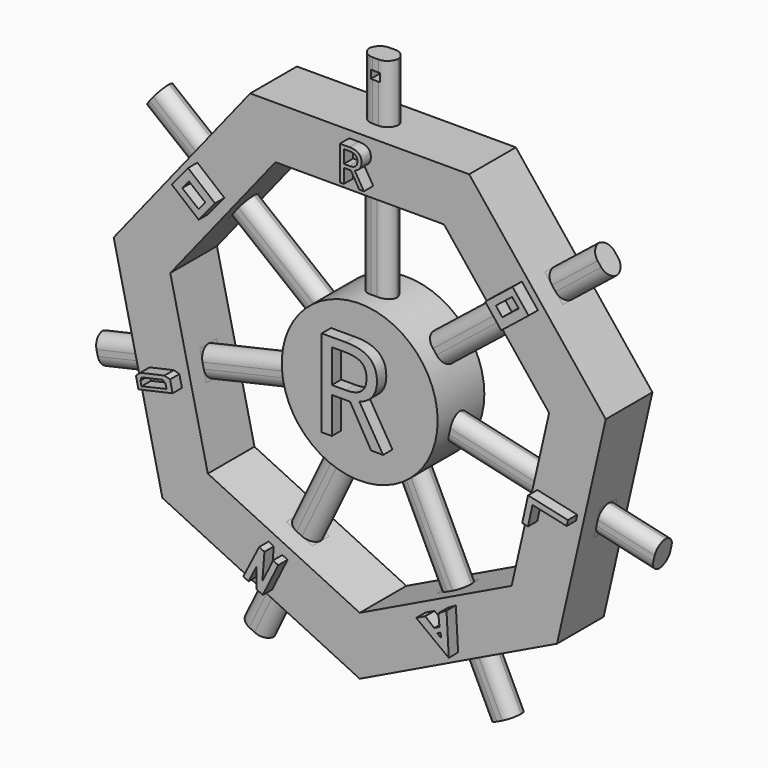
from build123d import *

# Parameters (mm, degrees)
F1_DEPTH      = 12.7
F7_W          = 6.35
F7_H          = 4.572
F9_DEPTH      = 25.4
F2_W          = 4.572
F2_H          = 6.35
F10_DEPTH     = 25.4
F4_W          = 6.35
F4_H          = 4.572
F11_DEPTH     = 25.4
F6_W          = 4.572
F6_H          = 6.35
F12_DEPTH     = 25.4
F3_W          = 6.35
F3_H          = 4.572
F13_DEPTH     = 25.4
F5_W          = 4.572
F5_H          = 6.35
F14_DEPTH     = 25.4
F8_W          = 4.572
F8_H          = 6.35
F15_DEPTH     = 25.4
F16_R         = 16.968135236
F17_DEPTH     = 12.7
F18_T4_DEPTH  = 27.8007641953
F18_S5_R      = 16.968135236
F18_T6_DEPTH  = 16
F18_T10_DEPTH = 27.7765131314
F18_S11_R     = 16.968135236
F18_T12_DEPTH = 16
F18_T16_DEPTH = 27.7765131314
F18_S17_R     = 16.968135236
F18_T18_DEPTH = 16
F18_T22_DEPTH = 27.8007641953
F18_S23_R     = 16.968135236
F18_T24_DEPTH = 16
F19_T4_DEPTH  = 27.7765131314
F19_S5_R      = 16.968135236
F19_T6_DEPTH  = 17
F19_T10_DEPTH = 27.8007641953
F19_S11_R     = 16.968135236
F19_T12_DEPTH = 17
F19_T16_DEPTH = 27.8007641953
F19_S17_R     = 16.968135236
F19_T18_DEPTH = 17
F19_T22_DEPTH = 27.7765131314
F19_S23_R     = 16.968135236
F19_T24_DEPTH = 17
F20_T4_DEPTH  = 27.7765131314
F20_S5_R      = 16.968135236
F20_T6_DEPTH  = 16
F20_T10_DEPTH = 27.8007641953
F20_S11_R     = 16.968135236
F20_T12_DEPTH = 16
F20_T16_DEPTH = 27.8007641953
F20_S17_R     = 16.968135236
F20_T18_DEPTH = 16
F20_T22_DEPTH = 27.7765131314
F20_S23_R     = 16.968135236
F20_T24_DEPTH = 16
F21_T4_DEPTH  = 27.8007641953
F21_S5_R      = 16.968135236
F21_T6_DEPTH  = 17
F21_T10_DEPTH = 27.7765131314
F21_S11_R     = 16.968135236
F21_T12_DEPTH = 17
F21_T16_DEPTH = 27.8007641953
F21_S17_R     = 16.968135236
F21_T18_DEPTH = 17
F21_T22_DEPTH = 27.7765131314
F21_S23_R     = 16.968135236
F21_T24_DEPTH = 17
F22_T4_DEPTH  = 27.8007641953
F22_S5_R      = 16.968135236
F22_T6_DEPTH  = 16
F22_T10_DEPTH = 27.7765131314
F22_S11_R     = 16.968135236
F22_T12_DEPTH = 16
F22_T16_DEPTH = 27.7765131314
F22_S17_R     = 16.968135236
F22_T18_DEPTH = 16
F22_T22_DEPTH = 27.8007641953
F22_S23_R     = 16.968135236
F22_T24_DEPTH = 16
F23_T4_DEPTH  = 27.8007641953
F23_S5_R      = 16.968135236
F23_T6_DEPTH  = 16
F23_T10_DEPTH = 27.7765131314
F23_S11_R     = 16.968135236
F23_T12_DEPTH = 16
F23_T16_DEPTH = 27.7765131314
F23_S17_R     = 16.968135236
F23_T18_DEPTH = 16
F23_T22_DEPTH = 27.8007641953
F23_S23_R     = 16.968135236
F23_T24_DEPTH = 16
F24_T4_DEPTH  = 27.8007641953
F24_S5_R      = 16.968135236
F24_T6_DEPTH  = 16
F24_T10_DEPTH = 27.7765131314
F24_S11_R     = 16.968135236
F24_T12_DEPTH = 16
F24_T16_DEPTH = 27.8007641953
F24_S17_R     = 16.968135236
F24_T18_DEPTH = 16
F24_T22_DEPTH = 27.7765131314
F24_S23_R     = 16.968135236
F24_T24_DEPTH = 16
F25_W         = 4.572
F25_H         = 6.35
F26_DEPTH     = 12.7
F32_W         = 4.572
F32_H         = 6.35
F33_DEPTH     = 12.7
F31_W         = 6.35
F31_H         = 4.572
F34_DEPTH     = 12.7
F30_W         = 4.572
F30_H         = 6.35
F35_DEPTH     = 12.7
F29_W         = 4.572
F29_H         = 6.35
F36_DEPTH     = 12.7
F28_W         = 6.35
F28_H         = 4.572
F37_DEPTH     = 12.7
F27_W         = 6.35
F27_H         = 4.572
F38_DEPTH     = 12.7
F39_T1_DEPTH  = 19.05
F40_T1_DEPTH  = 19.05
F41_T1_DEPTH  = 19.05
F42_T1_DEPTH  = 19.05
F43_T1_DEPTH  = 19.05
F44_T1_DEPTH  = 19.05
F45_T1_DEPTH  = 19.05
F46_W         = 0.3858066193
F46_H         = 1.778
F46_W_2       = 1.27
F46_W_3       = 0.3761933807
F47_DEPTH     = 25.4
F48_TEXT_SIZE = 26.5507492438
F49_DEPTH     = 2.54
F50_TEXT_SIZE = 26.5466622973
F51_DEPTH     = 2.54
F52_TEXT_SIZE = 10.4224828589
F53_DEPTH     = 2.54


# Not quite as in the source:
# - a fillet or chamfer that OpenCascade refuses, or shapes differently, is made with other operations: its cross-section is extruded or revolved along the edge and cut away or added
# - Text() gives the source's letters only with a copy of the font that has no kerning and outlines rounded to 1/6400 em; it was checked with that copy


with BuildPart() as f1:
    # F0 (on Front) → F1 (new body)
    with BuildSketch(Plane.XZ):
        Polygon((23.8356489691, 49.4952350855), (-23.8356489691, 49.4952350855), (-53.5582170749, 12.2243135473), (-42.9503553348, -34.2517654225), (0, -54.9355664205), (42.9503553348, -34.2517654225), (53.5582170749, 12.2243135473), align=None)
        Polygon((-41.2350925481, 9.41164079), (-18.3513426111, 38.1069555879), (18.3513426111, 38.1069555879), (41.2350925481, 9.41164079), (33.0679767537, -26.3708314853), (0, -42.2955297852), (-33.0679767537, -26.3708314853), align=None, mode=Mode.SUBTRACT)
    extrude(amount=F1_DEPTH)

    # F7 (on face) → F9 (join)
    with BuildSketch(Plane(origin=(0, 0, 38.1069555879), x_dir=(1, 0, 0), z_dir=(0, 0, -1))):
        with Locations((0.0636573889, 6.604)):
            Rectangle(F7_W, F7_H)
    extrude(amount=F9_DEPTH)

    # F2 (on face) → F10 (join)
    with BuildSketch(Plane(origin=(-37.1515346509, 0, -8.4795953476), x_dir=(0, 1, 0), z_dir=(0.9749279122, 0, 0.222520934))):
        with Locations((-6.604, -0.0636573889)):
            Rectangle(F2_W, F2_H)
    extrude(amount=F10_DEPTH)

    # F4 (on face) → F11 (join)
    with BuildSketch(Plane(origin=(16.5339883768, 0, -34.3331806352), x_dir=(0.9009688679, 0, 0.4338837391), z_dir=(-0.4338837391, 0, 0.9009688679))):
        with Locations((0.0636573889, -6.604)):
            Rectangle(F4_W, F4_H)
    extrude(amount=F11_DEPTH)

    # F6 (on face) → F12 (join)
    with BuildSketch(Plane(origin=(29.7932175796, 0, 23.7592981889), x_dir=(0, -1, 0), z_dir=(-0.7818314825, 0, -0.6234898019))):
        with Locations((6.604, -0.0636573889)):
            Rectangle(F6_W, F6_H)
    extrude(amount=F12_DEPTH)

    # F3 (on face) → F13 (join)
    with BuildSketch(Plane(origin=(-16.5339883768, 0, -34.3331806352), x_dir=(0.9009688679, 0, -0.4338837391), z_dir=(0.4338837391, 0, 0.9009688679))):
        with Locations((-0.0636573889, -6.096)):
            Rectangle(F3_W, F3_H)
    extrude(amount=F13_DEPTH)

    # F5 (on face) → F14 (join)
    with BuildSketch(Plane(origin=(37.1515346509, 0, -8.4795953476), x_dir=(0, -1, 0), z_dir=(-0.9749279122, 0, 0.222520934))):
        with Locations((6.604, 0.0636573889)):
            Rectangle(F5_W, F5_H)
    extrude(amount=F14_DEPTH)

    # F8 (on face) → F15 (join)
    with BuildSketch(Plane(origin=(-29.7932175796, 0, 23.7592981889), x_dir=(0, 1, 0), z_dir=(0.7818314825, 0, -0.6234898019))):
        with Locations((-6.604, -0.0636573889)):
            Rectangle(F8_W, F8_H)
    extrude(amount=F15_DEPTH)

    # F16 (on Front) → F17 (join)
    with BuildSketch(Plane.XZ):
        Circle(F16_R)
    extrude(amount=F17_DEPTH)

    # F18: fillet of radius 2.54 on 4 edges, made by hand


with BuildPart() as f18_tool2:
    # F18_s3 → F18_t4 (new body)
    with BuildSketch(Plane(origin=(37.1515346509, 0, -8.4795953476), x_dir=(0, 1, 0), z_dir=(-0.9749279122, 0, 0.222520934))):
        with BuildLine():
            ThreePointArc((-6.35, -3.2386573889), (-8.1460512242, -2.4947086131), (-8.89, -0.6986573889))
            Line((-8.89, -0.6986573889), (-8.89, -3.2386573889))
            Line((-8.89, -3.2386573889), (-6.35, -3.2386573889))
        make_face()
    extrude(amount=F18_T4_DEPTH)

    # F18_s5 → F18_t6 (cut, symmetric)
    with BuildSketch(Plane.XZ.offset(7.6)):
        Circle(F18_S5_R)
    extrude(amount=F18_T6_DEPTH, both=True, mode=Mode.SUBTRACT)


with BuildPart() as f1_1:
    add(f1.part)

    # F18_t1: cut F18_tool2
    add(f18_tool2.part, mode=Mode.SUBTRACT)


with BuildPart() as f18_tool8:
    # F18_s9 → F18_t10 (new body)
    with BuildSketch(Plane(origin=(37.1515346509, 0, -8.4795953476), x_dir=(0, 1, 0), z_dir=(-0.9749279122, 0, 0.222520934))):
        with BuildLine():
            ThreePointArc((-4.318, 0.5713426111), (-5.0619487758, 2.3673938354), (-6.858, 3.1113426111))
            Line((-6.858, 3.1113426111), (-4.318, 3.1113426111))
            Line((-4.318, 3.1113426111), (-4.318, 0.5713426111))
        make_face()
    extrude(amount=F18_T10_DEPTH)

    # F18_s11 → F18_t12 (cut, symmetric)
    with BuildSketch(Plane.XZ.offset(5.6)):
        Circle(F18_S11_R)
    extrude(amount=F18_T12_DEPTH, both=True, mode=Mode.SUBTRACT)


with BuildPart() as f1_2:
    add(f1_1.part)

    # F18_t7: cut F18_tool8
    add(f18_tool8.part, mode=Mode.SUBTRACT)


with BuildPart() as f18_tool14:
    # F18_s15 → F18_t16 (new body)
    with BuildSketch(Plane(origin=(37.1515346509, 0, -8.4795953476), x_dir=(0, 1, 0), z_dir=(-0.9749279122, 0, 0.222520934))):
        with BuildLine():
            ThreePointArc((-8.89, 0.5713426111), (-8.1460512242, 2.3673938354), (-6.35, 3.1113426111))
            Line((-6.35, 3.1113426111), (-8.89, 3.1113426111))
            Line((-8.89, 3.1113426111), (-8.89, 0.5713426111))
        make_face()
    extrude(amount=F18_T16_DEPTH)

    # F18_s17 → F18_t18 (cut, symmetric)
    with BuildSketch(Plane.XZ.offset(7.6)):
        Circle(F18_S17_R)
    extrude(amount=F18_T18_DEPTH, both=True, mode=Mode.SUBTRACT)


with BuildPart() as f1_3:
    add(f1_2.part)

    # F18_t13: cut F18_tool14
    add(f18_tool14.part, mode=Mode.SUBTRACT)


with BuildPart() as f18_tool20:
    # F18_s21 → F18_t22 (new body)
    with BuildSketch(Plane(origin=(37.1515346509, 0, -8.4795953476), x_dir=(0, 1, 0), z_dir=(-0.9749279122, 0, 0.222520934))):
        with BuildLine():
            ThreePointArc((-4.318, -0.6986573889), (-5.0619487758, -2.4947086131), (-6.858, -3.2386573889))
            Line((-6.858, -3.2386573889), (-4.318, -3.2386573889))
            Line((-4.318, -3.2386573889), (-4.318, -0.6986573889))
        make_face()
    extrude(amount=F18_T22_DEPTH)

    # F18_s23 → F18_t24 (cut, symmetric)
    with BuildSketch(Plane.XZ.offset(5.6)):
        Circle(F18_S23_R)
    extrude(amount=F18_T24_DEPTH, both=True, mode=Mode.SUBTRACT)


with BuildPart() as f1_4:
    add(f1_3.part)

    # F18_t19: cut F18_tool20
    add(f18_tool20.part, mode=Mode.SUBTRACT)

    # F19: fillet of radius 2.54 on 4 edges, made by hand


with BuildPart() as f19_tool2:
    # F19_s3 → F19_t4 (new body)
    with BuildSketch(Plane(origin=(29.7932175796, 0, 23.7592981889), x_dir=(0, 1, 0), z_dir=(-0.7818314825, 0, -0.6234898019))):
        with BuildLine():
            ThreePointArc((-8.89, -0.5713426111), (-8.1460512242, -2.3673938354), (-6.35, -3.1113426111))
            Line((-6.35, -3.1113426111), (-8.89, -3.1113426111))
            Line((-8.89, -3.1113426111), (-8.89, -0.5713426111))
        make_face()
    extrude(amount=F19_T4_DEPTH)

    # F19_s5 → F19_t6 (cut, symmetric)
    with BuildSketch(Plane.XZ.offset(7.6)):
        Circle(F19_S5_R)
    extrude(amount=F19_T6_DEPTH, both=True, mode=Mode.SUBTRACT)


with BuildPart() as f1_5:
    add(f1_4.part)

    # F19_t1: cut F19_tool2
    add(f19_tool2.part, mode=Mode.SUBTRACT)


with BuildPart() as f19_tool8:
    # F19_s9 → F19_t10 (new body)
    with BuildSketch(Plane(origin=(29.7932175796, 0, 23.7592981889), x_dir=(0, 1, 0), z_dir=(-0.7818314825, 0, -0.6234898019))):
        with BuildLine():
            ThreePointArc((-6.35, 3.2386573889), (-8.1460512242, 2.4947086131), (-8.89, 0.6986573889))
            Line((-8.89, 0.6986573889), (-8.89, 3.2386573889))
            Line((-8.89, 3.2386573889), (-6.35, 3.2386573889))
        make_face()
    extrude(amount=F19_T10_DEPTH)

    # F19_s11 → F19_t12 (cut, symmetric)
    with BuildSketch(Plane.XZ.offset(7.6)):
        Circle(F19_S11_R)
    extrude(amount=F19_T12_DEPTH, both=True, mode=Mode.SUBTRACT)


with BuildPart() as f1_6:
    add(f1_5.part)

    # F19_t7: cut F19_tool8
    add(f19_tool8.part, mode=Mode.SUBTRACT)


with BuildPart() as f19_tool14:
    # F19_s15 → F19_t16 (new body)
    with BuildSketch(Plane(origin=(29.7932175796, 0, 23.7592981889), x_dir=(0, 1, 0), z_dir=(-0.7818314825, 0, -0.6234898019))):
        with BuildLine():
            ThreePointArc((-4.318, 0.6986573889), (-5.0619487758, 2.4947086131), (-6.858, 3.2386573889))
            Line((-6.858, 3.2386573889), (-4.318, 3.2386573889))
            Line((-4.318, 3.2386573889), (-4.318, 0.6986573889))
        make_face()
    extrude(amount=F19_T16_DEPTH)

    # F19_s17 → F19_t18 (cut, symmetric)
    with BuildSketch(Plane.XZ.offset(5.6)):
        Circle(F19_S17_R)
    extrude(amount=F19_T18_DEPTH, both=True, mode=Mode.SUBTRACT)


with BuildPart() as f1_7:
    add(f1_6.part)

    # F19_t13: cut F19_tool14
    add(f19_tool14.part, mode=Mode.SUBTRACT)


with BuildPart() as f19_tool20:
    # F19_s21 → F19_t22 (new body)
    with BuildSketch(Plane(origin=(29.7932175796, 0, 23.7592981889), x_dir=(0, 1, 0), z_dir=(-0.7818314825, 0, -0.6234898019))):
        with BuildLine():
            ThreePointArc((-4.318, -0.5713426111), (-5.0619487758, -2.3673938354), (-6.858, -3.1113426111))
            Line((-6.858, -3.1113426111), (-4.318, -3.1113426111))
            Line((-4.318, -3.1113426111), (-4.318, -0.5713426111))
        make_face()
    extrude(amount=F19_T22_DEPTH)

    # F19_s23 → F19_t24 (cut, symmetric)
    with BuildSketch(Plane.XZ.offset(5.6)):
        Circle(F19_S23_R)
    extrude(amount=F19_T24_DEPTH, both=True, mode=Mode.SUBTRACT)


with BuildPart() as f1_8:
    add(f1_7.part)

    # F19_t19: cut F19_tool20
    add(f19_tool20.part, mode=Mode.SUBTRACT)

    # F20: fillet of radius 2.54 on 4 edges, made by hand


with BuildPart() as f20_tool2:
    # F20_s3 → F20_t4 (new body)
    with BuildSketch(Plane.XY.offset(38.1069555879)):
        with BuildLine():
            ThreePointArc((-0.5713426111, -8.89), (-2.3673938354, -8.1460512242), (-3.1113426111, -6.35))
            Line((-3.1113426111, -6.35), (-3.1113426111, -8.89))
            Line((-3.1113426111, -8.89), (-0.5713426111, -8.89))
        make_face()
    extrude(amount=-F20_T4_DEPTH)

    # F20_s5 → F20_t6 (cut, symmetric)
    with BuildSketch(Plane.XZ.offset(7.6)):
        Circle(F20_S5_R)
    extrude(amount=F20_T6_DEPTH, both=True, mode=Mode.SUBTRACT)


with BuildPart() as f1_9:
    add(f1_8.part)

    # F20_t1: cut F20_tool2
    add(f20_tool2.part, mode=Mode.SUBTRACT)


with BuildPart() as f20_tool8:
    # F20_s9 → F20_t10 (new body)
    with BuildSketch(Plane.XY.offset(38.1069555879)):
        with BuildLine():
            ThreePointArc((0.6986573889, -4.318), (2.4947086131, -5.0619487758), (3.2386573889, -6.858))
            Line((3.2386573889, -6.858), (3.2386573889, -4.318))
            Line((3.2386573889, -4.318), (0.6986573889, -4.318))
        make_face()
    extrude(amount=-F20_T10_DEPTH)

    # F20_s11 → F20_t12 (cut, symmetric)
    with BuildSketch(Plane.XZ.offset(5.6)):
        Circle(F20_S11_R)
    extrude(amount=F20_T12_DEPTH, both=True, mode=Mode.SUBTRACT)


with BuildPart() as f1_10:
    add(f1_9.part)

    # F20_t7: cut F20_tool8
    add(f20_tool8.part, mode=Mode.SUBTRACT)


with BuildPart() as f20_tool14:
    # F20_s15 → F20_t16 (new body)
    with BuildSketch(Plane.XY.offset(38.1069555879)):
        with BuildLine():
            ThreePointArc((3.2386573889, -6.35), (2.4947086131, -8.1460512242), (0.6986573889, -8.89))
            Line((0.6986573889, -8.89), (3.2386573889, -8.89))
            Line((3.2386573889, -8.89), (3.2386573889, -6.35))
        make_face()
    extrude(amount=-F20_T16_DEPTH)

    # F20_s17 → F20_t18 (cut, symmetric)
    with BuildSketch(Plane.XZ.offset(7.6)):
        Circle(F20_S17_R)
    extrude(amount=F20_T18_DEPTH, both=True, mode=Mode.SUBTRACT)


with BuildPart() as f1_11:
    add(f1_10.part)

    # F20_t13: cut F20_tool14
    add(f20_tool14.part, mode=Mode.SUBTRACT)


with BuildPart() as f20_tool20:
    # F20_s21 → F20_t22 (new body)
    with BuildSketch(Plane.XY.offset(38.1069555879)):
        with BuildLine():
            ThreePointArc((-0.5713426111, -4.318), (-2.3673938354, -5.0619487758), (-3.1113426111, -6.858))
            Line((-3.1113426111, -6.858), (-3.1113426111, -4.318))
            Line((-3.1113426111, -4.318), (-0.5713426111, -4.318))
        make_face()
    extrude(amount=-F20_T22_DEPTH)

    # F20_s23 → F20_t24 (cut, symmetric)
    with BuildSketch(Plane.XZ.offset(5.6)):
        Circle(F20_S23_R)
    extrude(amount=F20_T24_DEPTH, both=True, mode=Mode.SUBTRACT)


with BuildPart() as f1_12:
    add(f1_11.part)

    # F20_t19: cut F20_tool20
    add(f20_tool20.part, mode=Mode.SUBTRACT)

    # F21: fillet of radius 2.54 on 4 edges, made by hand


with BuildPart() as f21_tool2:
    # F21_s3 → F21_t4 (new body)
    with BuildSketch(Plane(origin=(-29.7932175796, 0, 23.7592981889), x_dir=(0, 1, 0), z_dir=(0.7818314825, 0, -0.6234898019))):
        with BuildLine():
            ThreePointArc((-4.318, -0.6986573889), (-5.0619487758, -2.4947086131), (-6.858, -3.2386573889))
            Line((-6.858, -3.2386573889), (-4.318, -3.2386573889))
            Line((-4.318, -3.2386573889), (-4.318, -0.6986573889))
        make_face()
    extrude(amount=F21_T4_DEPTH)

    # F21_s5 → F21_t6 (cut, symmetric)
    with BuildSketch(Plane.XZ.offset(5.6)):
        Circle(F21_S5_R)
    extrude(amount=F21_T6_DEPTH, both=True, mode=Mode.SUBTRACT)


with BuildPart() as f1_13:
    add(f1_12.part)

    # F21_t1: cut F21_tool2
    add(f21_tool2.part, mode=Mode.SUBTRACT)


with BuildPart() as f21_tool8:
    # F21_s9 → F21_t10 (new body)
    with BuildSketch(Plane(origin=(-29.7932175796, 0, 23.7592981889), x_dir=(0, 1, 0), z_dir=(0.7818314825, 0, -0.6234898019))):
        with BuildLine():
            ThreePointArc((-4.318, 0.5713426111), (-5.0619487758, 2.3673938354), (-6.858, 3.1113426111))
            Line((-6.858, 3.1113426111), (-4.318, 3.1113426111))
            Line((-4.318, 3.1113426111), (-4.318, 0.5713426111))
        make_face()
    extrude(amount=F21_T10_DEPTH)

    # F21_s11 → F21_t12 (cut, symmetric)
    with BuildSketch(Plane.XZ.offset(5.6)):
        Circle(F21_S11_R)
    extrude(amount=F21_T12_DEPTH, both=True, mode=Mode.SUBTRACT)


with BuildPart() as f1_14:
    add(f1_13.part)

    # F21_t7: cut F21_tool8
    add(f21_tool8.part, mode=Mode.SUBTRACT)


with BuildPart() as f21_tool14:
    # F21_s15 → F21_t16 (new body)
    with BuildSketch(Plane(origin=(-29.7932175796, 0, 23.7592981889), x_dir=(0, 1, 0), z_dir=(0.7818314825, 0, -0.6234898019))):
        with BuildLine():
            ThreePointArc((-8.89, -0.6986573889), (-8.1460512242, -2.4947086131), (-6.35, -3.2386573889))
            Line((-6.35, -3.2386573889), (-8.89, -3.2386573889))
            Line((-8.89, -3.2386573889), (-8.89, -0.6986573889))
        make_face()
    extrude(amount=F21_T16_DEPTH)

    # F21_s17 → F21_t18 (cut, symmetric)
    with BuildSketch(Plane.XZ.offset(7.6)):
        Circle(F21_S17_R)
    extrude(amount=F21_T18_DEPTH, both=True, mode=Mode.SUBTRACT)


with BuildPart() as f1_15:
    add(f1_14.part)

    # F21_t13: cut F21_tool14
    add(f21_tool14.part, mode=Mode.SUBTRACT)


with BuildPart() as f21_tool20:
    # F21_s21 → F21_t22 (new body)
    with BuildSketch(Plane(origin=(-29.7932175796, 0, 23.7592981889), x_dir=(0, 1, 0), z_dir=(0.7818314825, 0, -0.6234898019))):
        with BuildLine():
            ThreePointArc((-6.35, 3.1113426111), (-8.1460512242, 2.3673938354), (-8.89, 0.5713426111))
            Line((-8.89, 0.5713426111), (-8.89, 3.1113426111))
            Line((-8.89, 3.1113426111), (-6.35, 3.1113426111))
        make_face()
    extrude(amount=F21_T22_DEPTH)

    # F21_s23 → F21_t24 (cut, symmetric)
    with BuildSketch(Plane.XZ.offset(7.6)):
        Circle(F21_S23_R)
    extrude(amount=F21_T24_DEPTH, both=True, mode=Mode.SUBTRACT)


with BuildPart() as f1_16:
    add(f1_15.part)

    # F21_t19: cut F21_tool20
    add(f21_tool20.part, mode=Mode.SUBTRACT)

    # F22: fillet of radius 2.54 on 4 edges, made by hand


with BuildPart() as f22_tool2:
    # F22_s3 → F22_t4 (new body)
    with BuildSketch(Plane(origin=(-37.1515346509, 0, -8.4795953476), x_dir=(0, 1, 0), z_dir=(0.9749279122, 0, 0.222520934))):
        with BuildLine():
            ThreePointArc((-4.318, -0.6986573889), (-5.0619487758, -2.4947086131), (-6.858, -3.2386573889))
            Line((-6.858, -3.2386573889), (-4.318, -3.2386573889))
            Line((-4.318, -3.2386573889), (-4.318, -0.6986573889))
        make_face()
    extrude(amount=F22_T4_DEPTH)

    # F22_s5 → F22_t6 (cut, symmetric)
    with BuildSketch(Plane.XZ.offset(5.6)):
        Circle(F22_S5_R)
    extrude(amount=F22_T6_DEPTH, both=True, mode=Mode.SUBTRACT)


with BuildPart() as f1_17:
    add(f1_16.part)

    # F22_t1: cut F22_tool2
    add(f22_tool2.part, mode=Mode.SUBTRACT)


with BuildPart() as f22_tool8:
    # F22_s9 → F22_t10 (new body)
    with BuildSketch(Plane(origin=(-37.1515346509, 0, -8.4795953476), x_dir=(0, 1, 0), z_dir=(0.9749279122, 0, 0.222520934))):
        with BuildLine():
            ThreePointArc((-4.318, 0.5713426111), (-5.0619487758, 2.3673938354), (-6.858, 3.1113426111))
            Line((-6.858, 3.1113426111), (-4.318, 3.1113426111))
            Line((-4.318, 3.1113426111), (-4.318, 0.5713426111))
        make_face()
    extrude(amount=F22_T10_DEPTH)

    # F22_s11 → F22_t12 (cut, symmetric)
    with BuildSketch(Plane.XZ.offset(5.6)):
        Circle(F22_S11_R)
    extrude(amount=F22_T12_DEPTH, both=True, mode=Mode.SUBTRACT)


with BuildPart() as f1_18:
    add(f1_17.part)

    # F22_t7: cut F22_tool8
    add(f22_tool8.part, mode=Mode.SUBTRACT)


with BuildPart() as f22_tool14:
    # F22_s15 → F22_t16 (new body)
    with BuildSketch(Plane(origin=(-37.1515346509, 0, -8.4795953476), x_dir=(0, 1, 0), z_dir=(0.9749279122, 0, 0.222520934))):
        with BuildLine():
            ThreePointArc((-8.89, 0.5713426111), (-8.1460512242, 2.3673938354), (-6.35, 3.1113426111))
            Line((-6.35, 3.1113426111), (-8.89, 3.1113426111))
            Line((-8.89, 3.1113426111), (-8.89, 0.5713426111))
        make_face()
    extrude(amount=F22_T16_DEPTH)

    # F22_s17 → F22_t18 (cut, symmetric)
    with BuildSketch(Plane.XZ.offset(7.6)):
        Circle(F22_S17_R)
    extrude(amount=F22_T18_DEPTH, both=True, mode=Mode.SUBTRACT)


with BuildPart() as f1_19:
    add(f1_18.part)

    # F22_t13: cut F22_tool14
    add(f22_tool14.part, mode=Mode.SUBTRACT)


with BuildPart() as f22_tool20:
    # F22_s21 → F22_t22 (new body)
    with BuildSketch(Plane(origin=(-37.1515346509, 0, -8.4795953476), x_dir=(0, 1, 0), z_dir=(0.9749279122, 0, 0.222520934))):
        with BuildLine():
            ThreePointArc((-6.35, -3.2386573889), (-8.1460512242, -2.4947086131), (-8.89, -0.6986573889))
            Line((-8.89, -0.6986573889), (-8.89, -3.2386573889))
            Line((-8.89, -3.2386573889), (-6.35, -3.2386573889))
        make_face()
    extrude(amount=F22_T22_DEPTH)

    # F22_s23 → F22_t24 (cut, symmetric)
    with BuildSketch(Plane.XZ.offset(7.6)):
        Circle(F22_S23_R)
    extrude(amount=F22_T24_DEPTH, both=True, mode=Mode.SUBTRACT)


with BuildPart() as f1_20:
    add(f1_19.part)

    # F22_t19: cut F22_tool20
    add(f22_tool20.part, mode=Mode.SUBTRACT)

    # F23: fillet of radius 2.54 on 4 edges, made by hand


with BuildPart() as f23_tool2:
    # F23_s3 → F23_t4 (new body)
    with BuildSketch(Plane(origin=(-16.5339883768, 0, -34.3331806352), x_dir=(0, 1, 0), z_dir=(0.4338837391, 0, 0.9009688679))):
        with BuildLine():
            ThreePointArc((-6.35, 3.2386573889), (-4.5539487758, 2.4947086131), (-3.81, 0.6986573889))
            Line((-3.81, 0.6986573889), (-3.81, 3.2386573889))
            Line((-3.81, 3.2386573889), (-6.35, 3.2386573889))
        make_face()
    extrude(amount=F23_T4_DEPTH)

    # F23_s5 → F23_t6 (cut, symmetric)
    with BuildSketch(Plane.XZ.offset(5.1)):
        Circle(F23_S5_R)
    extrude(amount=F23_T6_DEPTH, both=True, mode=Mode.SUBTRACT)


with BuildPart() as f1_21:
    add(f1_20.part)

    # F23_t1: cut F23_tool2
    add(f23_tool2.part, mode=Mode.SUBTRACT)


with BuildPart() as f23_tool8:
    # F23_s9 → F23_t10 (new body)
    with BuildSketch(Plane(origin=(-16.5339883768, 0, -34.3331806352), x_dir=(0, 1, 0), z_dir=(0.4338837391, 0, 0.9009688679))):
        with BuildLine():
            ThreePointArc((-6.35, -3.1113426111), (-4.5539487758, -2.3673938354), (-3.81, -0.5713426111))
            Line((-3.81, -0.5713426111), (-3.81, -3.1113426111))
            Line((-3.81, -3.1113426111), (-6.35, -3.1113426111))
        make_face()
    extrude(amount=F23_T10_DEPTH)

    # F23_s11 → F23_t12 (cut, symmetric)
    with BuildSketch(Plane.XZ.offset(5.1)):
        Circle(F23_S11_R)
    extrude(amount=F23_T12_DEPTH, both=True, mode=Mode.SUBTRACT)


with BuildPart() as f1_22:
    add(f1_21.part)

    # F23_t7: cut F23_tool8
    add(f23_tool8.part, mode=Mode.SUBTRACT)


with BuildPart() as f23_tool14:
    # F23_s15 → F23_t16 (new body)
    with BuildSketch(Plane(origin=(-16.5339883768, 0, -34.3331806352), x_dir=(0, 1, 0), z_dir=(0.4338837391, 0, 0.9009688679))):
        with BuildLine():
            ThreePointArc((-8.382, -0.5713426111), (-7.6380512242, -2.3673938354), (-5.842, -3.1113426111))
            Line((-5.842, -3.1113426111), (-8.382, -3.1113426111))
            Line((-8.382, -3.1113426111), (-8.382, -0.5713426111))
        make_face()
    extrude(amount=F23_T16_DEPTH)

    # F23_s17 → F23_t18 (cut, symmetric)
    with BuildSketch(Plane.XZ.offset(7.1)):
        Circle(F23_S17_R)
    extrude(amount=F23_T18_DEPTH, both=True, mode=Mode.SUBTRACT)


with BuildPart() as f1_23:
    add(f1_22.part)

    # F23_t13: cut F23_tool14
    add(f23_tool14.part, mode=Mode.SUBTRACT)


with BuildPart() as f23_tool20:
    # F23_s21 → F23_t22 (new body)
    with BuildSketch(Plane(origin=(-16.5339883768, 0, -34.3331806352), x_dir=(0, 1, 0), z_dir=(0.4338837391, 0, 0.9009688679))):
        with BuildLine():
            ThreePointArc((-5.842, 3.2386573889), (-7.6380512242, 2.4947086131), (-8.382, 0.6986573889))
            Line((-8.382, 0.6986573889), (-8.382, 3.2386573889))
            Line((-8.382, 3.2386573889), (-5.842, 3.2386573889))
        make_face()
    extrude(amount=F23_T22_DEPTH)

    # F23_s23 → F23_t24 (cut, symmetric)
    with BuildSketch(Plane.XZ.offset(7.1)):
        Circle(F23_S23_R)
    extrude(amount=F23_T24_DEPTH, both=True, mode=Mode.SUBTRACT)


with BuildPart() as f1_24:
    add(f1_23.part)

    # F23_t19: cut F23_tool20
    add(f23_tool20.part, mode=Mode.SUBTRACT)

    # F24: fillet of radius 2.54 on 4 edges, made by hand


with BuildPart() as f24_tool2:
    # F24_s3 → F24_t4 (new body)
    with BuildSketch(Plane(origin=(16.5339883768, 0, -34.3331806352), x_dir=(0, 1, 0), z_dir=(-0.4338837391, 0, 0.9009688679))):
        with BuildLine():
            ThreePointArc((-6.858, -3.2386573889), (-5.0619487758, -2.4947086131), (-4.318, -0.6986573889))
            Line((-4.318, -0.6986573889), (-4.318, -3.2386573889))
            Line((-4.318, -3.2386573889), (-6.858, -3.2386573889))
        make_face()
    extrude(amount=F24_T4_DEPTH)

    # F24_s5 → F24_t6 (cut, symmetric)
    with BuildSketch(Plane.XZ.offset(5.6)):
        Circle(F24_S5_R)
    extrude(amount=F24_T6_DEPTH, both=True, mode=Mode.SUBTRACT)


with BuildPart() as f1_25:
    add(f1_24.part)

    # F24_t1: cut F24_tool2
    add(f24_tool2.part, mode=Mode.SUBTRACT)


with BuildPart() as f24_tool8:
    # F24_s9 → F24_t10 (new body)
    with BuildSketch(Plane(origin=(16.5339883768, 0, -34.3331806352), x_dir=(0, 1, 0), z_dir=(-0.4338837391, 0, 0.9009688679))):
        with BuildLine():
            ThreePointArc((-6.858, 3.1113426111), (-5.0619487758, 2.3673938354), (-4.318, 0.5713426111))
            Line((-4.318, 0.5713426111), (-4.318, 3.1113426111))
            Line((-4.318, 3.1113426111), (-6.858, 3.1113426111))
        make_face()
    extrude(amount=F24_T10_DEPTH)

    # F24_s11 → F24_t12 (cut, symmetric)
    with BuildSketch(Plane.XZ.offset(5.6)):
        Circle(F24_S11_R)
    extrude(amount=F24_T12_DEPTH, both=True, mode=Mode.SUBTRACT)


with BuildPart() as f1_26:
    add(f1_25.part)

    # F24_t7: cut F24_tool8
    add(f24_tool8.part, mode=Mode.SUBTRACT)


with BuildPart() as f24_tool14:
    # F24_s15 → F24_t16 (new body)
    with BuildSketch(Plane(origin=(16.5339883768, 0, -34.3331806352), x_dir=(0, 1, 0), z_dir=(-0.4338837391, 0, 0.9009688679))):
        with BuildLine():
            ThreePointArc((-6.35, -3.2386573889), (-8.1460512242, -2.4947086131), (-8.89, -0.6986573889))
            Line((-8.89, -0.6986573889), (-8.89, -3.2386573889))
            Line((-8.89, -3.2386573889), (-6.35, -3.2386573889))
        make_face()
    extrude(amount=F24_T16_DEPTH)

    # F24_s17 → F24_t18 (cut, symmetric)
    with BuildSketch(Plane.XZ.offset(7.6)):
        Circle(F24_S17_R)
    extrude(amount=F24_T18_DEPTH, both=True, mode=Mode.SUBTRACT)


with BuildPart() as f1_27:
    add(f1_26.part)

    # F24_t13: cut F24_tool14
    add(f24_tool14.part, mode=Mode.SUBTRACT)


with BuildPart() as f24_tool20:
    # F24_s21 → F24_t22 (new body)
    with BuildSketch(Plane(origin=(16.5339883768, 0, -34.3331806352), x_dir=(0, 1, 0), z_dir=(-0.4338837391, 0, 0.9009688679))):
        with BuildLine():
            ThreePointArc((-8.89, 0.5713426111), (-8.1460512242, 2.3673938354), (-6.35, 3.1113426111))
            Line((-6.35, 3.1113426111), (-8.89, 3.1113426111))
            Line((-8.89, 3.1113426111), (-8.89, 0.5713426111))
        make_face()
    extrude(amount=F24_T22_DEPTH)

    # F24_s23 → F24_t24 (cut, symmetric)
    with BuildSketch(Plane.XZ.offset(7.6)):
        Circle(F24_S23_R)
    extrude(amount=F24_T24_DEPTH, both=True, mode=Mode.SUBTRACT)


with BuildPart() as f1_28:
    add(f1_27.part)

    # F24_t19: cut F24_tool20
    add(f24_tool20.part, mode=Mode.SUBTRACT)

    # F25 (on face) → F26 (join)
    with BuildSketch(Plane(origin=(-48.2542862048, 0, -11.0137259376), x_dir=(0, -1, 0), z_dir=(-0.9749279122, 0, -0.222520934))):
        with Locations((6.096, -0.12286896)):
            Rectangle(F25_W, F25_H)
    extrude(amount=F26_DEPTH)

    # F32 (on face) → F33 (join)
    with BuildSketch(Plane(origin=(-38.696933022, 0, 30.8597743164), x_dir=(0, -1, 0), z_dir=(-0.7818314825, 0, 0.6234898019))):
        with Locations((6.096, -0.2494668204)):
            Rectangle(F32_W, F32_H)
    extrude(amount=F33_DEPTH)

    # F31 (on face) → F34 (join)
    with BuildSketch(Plane.XY.offset(49.4952350855)):
        with Locations((-0.0392214861, -6.096)):
            Rectangle(F31_W, F31_H)
    extrude(amount=F34_DEPTH)

    # F30 (on face) → F35 (join)
    with BuildSketch(Plane(origin=(38.696933022, 0, 30.8597743164), x_dir=(0, 1, 0), z_dir=(0.7818314825, 0, 0.6234898019))):
        with Locations((-6.096, -0.1651499968)):
            Rectangle(F30_W, F30_H)
    extrude(amount=F35_DEPTH)

    # F29 (on face) → F36 (join)
    with BuildSketch(Plane(origin=(48.2542862048, 0, -11.0137259376), x_dir=(0, 1, 0), z_dir=(0.9749279122, 0, -0.222520934))):
        with Locations((-6.096, -0.073097375)):
            Rectangle(F29_W, F29_H)
    extrude(amount=F36_DEPTH)

    # F28 (on face) → F37 (join)
    with BuildSketch(Plane(origin=(21.4751776674, 0, -44.5936659215), x_dir=(0.9009688679, 0, 0.4338837391), z_dir=(0.4338837391, 0, -0.9009688679))):
        with Locations((0.0089227304, 6.096)):
            Rectangle(F28_W, F28_H)
    extrude(amount=F37_DEPTH)

    # F27 (on face) → F38 (join)
    with BuildSketch(Plane(origin=(-21.4751776674, 0, -44.5936659215), x_dir=(0.9009688679, 0, -0.4338837391), z_dir=(-0.4338837391, 0, -0.9009688679))):
        with Locations((0.0941157725, 6.096)):
            Rectangle(F27_W, F27_H)
    extrude(amount=F38_DEPTH)

    # F39: fillet of radius 2.54 on 4 edges, made by hand

    # F39_s2 → F39_t1 (cut)
    with BuildSketch(Plane(origin=(-48.2542862048, 0, -11.0137259376), x_dir=(0, 1, 0), z_dir=(-0.9749279122, 0, -0.222520934))):
        with BuildLine():
            ThreePointArc((-8.382, 0.75786896), (-7.6380512242, 2.5539201842), (-5.842, 3.29786896))
            Line((-5.842, 3.29786896), (-8.382, 3.29786896))
            Line((-8.382, 3.29786896), (-8.382, 0.75786896))
        make_face()
        with BuildLine():
            ThreePointArc((-5.842, -3.05213104), (-7.6380512242, -2.3081822642), (-8.382, -0.51213104))
            Line((-8.382, -0.51213104), (-8.382, -3.05213104))
            Line((-8.382, -3.05213104), (-5.842, -3.05213104))
        make_face()
        with BuildLine():
            ThreePointArc((-6.35, -3.05213104), (-4.5539487758, -2.3081822642), (-3.81, -0.51213104))
            Line((-3.81, -0.51213104), (-3.81, -3.05213104))
            Line((-3.81, -3.05213104), (-6.35, -3.05213104))
        make_face()
        with BuildLine():
            ThreePointArc((-6.35, 3.29786896), (-4.5539487758, 2.5539201842), (-3.81, 0.75786896))
            Line((-3.81, 0.75786896), (-3.81, 3.29786896))
            Line((-3.81, 3.29786896), (-6.35, 3.29786896))
        make_face()
    extrude(amount=F39_T1_DEPTH, mode=Mode.SUBTRACT)

    # F40: fillet of radius 2.54 on 4 edges, made by hand

    # F40_s2 → F40_t1 (cut)
    with BuildSketch(Plane(origin=(-21.4751776674, 0, -44.5936659215), x_dir=(0, 1, 0), z_dir=(-0.4338837391, 0, -0.9009688679))):
        with BuildLine():
            ThreePointArc((-5.842, 3.2691157725), (-7.6380512242, 2.5251669967), (-8.382, 0.7291157725))
            Line((-8.382, 0.7291157725), (-8.382, 3.2691157725))
            Line((-8.382, 3.2691157725), (-5.842, 3.2691157725))
        make_face()
        with BuildLine():
            ThreePointArc((-5.842, -3.0808842275), (-7.6380512242, -2.3369354517), (-8.382, -0.5408842275))
            Line((-8.382, -0.5408842275), (-8.382, -3.0808842275))
            Line((-8.382, -3.0808842275), (-5.842, -3.0808842275))
        make_face()
        with BuildLine():
            ThreePointArc((-6.35, 3.2691157725), (-4.5539487758, 2.5251669967), (-3.81, 0.7291157725))
            Line((-3.81, 0.7291157725), (-3.81, 3.2691157725))
            Line((-3.81, 3.2691157725), (-6.35, 3.2691157725))
        make_face()
        with BuildLine():
            ThreePointArc((-3.81, -0.5408842275), (-4.5539487758, -2.3369354517), (-6.35, -3.0808842275))
            Line((-6.35, -3.0808842275), (-3.81, -3.0808842275))
            Line((-3.81, -3.0808842275), (-3.81, -0.5408842275))
        make_face()
    extrude(amount=F40_T1_DEPTH, mode=Mode.SUBTRACT)

    # F41: fillet of radius 2.54 on 4 edges, made by hand

    # F41_s2 → F41_t1 (cut)
    with BuildSketch(Plane(origin=(21.4751776674, 0, -44.5936659215), x_dir=(0, 1, 0), z_dir=(0.4338837391, 0, -0.9009688679))):
        with BuildLine():
            ThreePointArc((-5.842, -3.1660772696), (-7.6380512242, -2.4221284938), (-8.382, -0.6260772696))
            Line((-8.382, -0.6260772696), (-8.382, -3.1660772696))
            Line((-8.382, -3.1660772696), (-5.842, -3.1660772696))
        make_face()
        with BuildLine():
            ThreePointArc((-8.382, 0.6439227304), (-7.6380512242, 2.4399739546), (-5.842, 3.1839227304))
            Line((-5.842, 3.1839227304), (-8.382, 3.1839227304))
            Line((-8.382, 3.1839227304), (-8.382, 0.6439227304))
        make_face()
        with BuildLine():
            ThreePointArc((-3.81, -0.6260772696), (-4.5539487758, -2.4221284938), (-6.35, -3.1660772696))
            Line((-6.35, -3.1660772696), (-3.81, -3.1660772696))
            Line((-3.81, -3.1660772696), (-3.81, -0.6260772696))
        make_face()
        with BuildLine():
            ThreePointArc((-3.81, 0.6439227304), (-4.5539487758, 2.4399739546), (-6.35, 3.1839227304))
            Line((-6.35, 3.1839227304), (-3.81, 3.1839227304))
            Line((-3.81, 3.1839227304), (-3.81, 0.6439227304))
        make_face()
    extrude(amount=F41_T1_DEPTH, mode=Mode.SUBTRACT)

    # F42: fillet of radius 2.54 on 4 edges, made by hand

    # F42_s2 → F42_t1 (cut)
    with BuildSketch(Plane(origin=(48.2542862048, 0, -11.0137259376), x_dir=(0, 1, 0), z_dir=(0.9749279122, 0, -0.222520934))):
        with BuildLine():
            ThreePointArc((-8.382, 0.561902625), (-7.6380512242, 2.3579538492), (-5.842, 3.101902625))
            Line((-5.842, 3.101902625), (-8.382, 3.101902625))
            Line((-8.382, 3.101902625), (-8.382, 0.561902625))
        make_face()
        with BuildLine():
            ThreePointArc((-5.842, -3.248097375), (-7.6380512242, -2.5041485992), (-8.382, -0.708097375))
            Line((-8.382, -0.708097375), (-8.382, -3.248097375))
            Line((-8.382, -3.248097375), (-5.842, -3.248097375))
        make_face()
        with BuildLine():
            ThreePointArc((-6.35, -3.248097375), (-4.5539487758, -2.5041485992), (-3.81, -0.708097375))
            Line((-3.81, -0.708097375), (-3.81, -3.248097375))
            Line((-3.81, -3.248097375), (-6.35, -3.248097375))
        make_face()
        with BuildLine():
            ThreePointArc((-6.35, 3.101902625), (-4.5539487758, 2.3579538492), (-3.81, 0.561902625))
            Line((-3.81, 0.561902625), (-3.81, 3.101902625))
            Line((-3.81, 3.101902625), (-6.35, 3.101902625))
        make_face()
    extrude(amount=F42_T1_DEPTH, mode=Mode.SUBTRACT)

    # F43: fillet of radius 2.54 on 4 edges, made by hand

    # F43_s2 → F43_t1 (cut)
    with BuildSketch(Plane(origin=(38.696933022, 0, 30.8597743164), x_dir=(0, 1, 0), z_dir=(0.7818314825, 0, 0.6234898019))):
        with BuildLine():
            ThreePointArc((-3.81, -0.8001499968), (-4.5539487758, -2.596201221), (-6.35, -3.3401499968))
            Line((-6.35, -3.3401499968), (-3.81, -3.3401499968))
            Line((-3.81, -3.3401499968), (-3.81, -0.8001499968))
        make_face()
        with BuildLine():
            ThreePointArc((-3.81, 0.4698500032), (-4.5539487758, 2.2659012274), (-6.35, 3.0098500032))
            Line((-6.35, 3.0098500032), (-3.81, 3.0098500032))
            Line((-3.81, 3.0098500032), (-3.81, 0.4698500032))
        make_face()
        with BuildLine():
            ThreePointArc((-8.382, 0.4698500032), (-7.6380512242, 2.2659012274), (-5.842, 3.0098500032))
            Line((-5.842, 3.0098500032), (-8.382, 3.0098500032))
            Line((-8.382, 3.0098500032), (-8.382, 0.4698500032))
        make_face()
        with BuildLine():
            ThreePointArc((-5.842, -3.3401499968), (-7.6380512242, -2.596201221), (-8.382, -0.8001499968))
            Line((-8.382, -0.8001499968), (-8.382, -3.3401499968))
            Line((-8.382, -3.3401499968), (-5.842, -3.3401499968))
        make_face()
    extrude(amount=F43_T1_DEPTH, mode=Mode.SUBTRACT)

    # F44: fillet of radius 2.54 on 4 edges, made by hand

    # F44_s2 → F44_t1 (cut)
    with BuildSketch(Plane(origin=(-38.696933022, 0, 30.8597743164), x_dir=(0, 1, 0), z_dir=(-0.7818314825, 0, 0.6234898019))):
        with BuildLine():
            ThreePointArc((-8.382, 0.8844668204), (-7.6380512242, 2.6805180446), (-5.842, 3.4244668204))
            Line((-5.842, 3.4244668204), (-8.382, 3.4244668204))
            Line((-8.382, 3.4244668204), (-8.382, 0.8844668204))
        make_face()
        with BuildLine():
            ThreePointArc((-5.842, -2.9255331796), (-7.6380512242, -2.1815844038), (-8.382, -0.3855331796))
            Line((-8.382, -0.3855331796), (-8.382, -2.9255331796))
            Line((-8.382, -2.9255331796), (-5.842, -2.9255331796))
        make_face()
        with BuildLine():
            ThreePointArc((-6.35, -2.9255331796), (-4.5539487758, -2.1815844038), (-3.81, -0.3855331796))
            Line((-3.81, -0.3855331796), (-3.81, -2.9255331796))
            Line((-3.81, -2.9255331796), (-6.35, -2.9255331796))
        make_face()
        with BuildLine():
            ThreePointArc((-6.35, 3.4244668204), (-4.5539487758, 2.6805180446), (-3.81, 0.8844668204))
            Line((-3.81, 0.8844668204), (-3.81, 3.4244668204))
            Line((-3.81, 3.4244668204), (-6.35, 3.4244668204))
        make_face()
    extrude(amount=F44_T1_DEPTH, mode=Mode.SUBTRACT)

    # F45: fillet of radius 2.54 on 4 edges, made by hand

    # F45_s2 → F45_t1 (cut)
    with BuildSketch(Plane.XY.offset(49.4952350855)):
        with BuildLine():
            ThreePointArc((0.5957785139, -3.81), (2.3918297381, -4.5539487758), (3.1357785139, -6.35))
            Line((3.1357785139, -6.35), (3.1357785139, -3.81))
            Line((3.1357785139, -3.81), (0.5957785139, -3.81))
        make_face()
        with BuildLine():
            ThreePointArc((-3.2142214861, -6.35), (-2.4702727103, -4.5539487758), (-0.6742214861, -3.81))
            Line((-0.6742214861, -3.81), (-3.2142214861, -3.81))
            Line((-3.2142214861, -3.81), (-3.2142214861, -6.35))
        make_face()
        with BuildLine():
            ThreePointArc((-0.6742214861, -8.382), (-2.4702727103, -7.6380512242), (-3.2142214861, -5.842))
            Line((-3.2142214861, -5.842), (-3.2142214861, -8.382))
            Line((-3.2142214861, -8.382), (-0.6742214861, -8.382))
        make_face()
        with BuildLine():
            ThreePointArc((0.5957785139, -8.382), (2.3918297381, -7.6380512242), (3.1357785139, -5.842))
            Line((3.1357785139, -5.842), (3.1357785139, -8.382))
            Line((3.1357785139, -8.382), (0.5957785139, -8.382))
        make_face()
    extrude(amount=F45_T1_DEPTH, mode=Mode.SUBTRACT)

    # F46 (on face) → F47 (cut)
    with BuildSketch(Plane(origin=(0, -3.81, 0), x_dir=(-1, 0, 0), z_dir=(0, 1, 0))):
        with Locations((-0.7886818236, 58.8244315996)):
            Rectangle(F46_W, F46_H)
        with Locations((0.0392214861, 58.8244315996)):
            Rectangle(F46_W_2, F46_H)
        with Locations((0.8623181764, 58.8244315996)):
            Rectangle(F46_W_3, F46_H)
    extrude(amount=-F47_DEPTH, mode=Mode.SUBTRACT)

    # F48 (on face) → F49 (join)
    with BuildSketch(Plane.XZ.offset(12.7)):
        with Locations((-8.8376310084, -8.6925512337)):
            Text('R', F48_TEXT_SIZE, font='Open Sans', text_align=(TextAlign.LEFT, TextAlign.BOTTOM))
    extrude(amount=F49_DEPTH)

    # F50 (on face) → F51 (join)
    with BuildSketch(Plane(origin=(0, 0, 0), x_dir=(-1, 0, 0), z_dir=(0, 1, 0))):
        with Locations((-8.8392089618, -8.6909466527)):
            Text('R', F50_TEXT_SIZE, font='Open Sans', text_align=(TextAlign.LEFT, TextAlign.BOTTOM))
    extrude(amount=F51_DEPTH)

    # F52 (on face) → F53 (join)
    with BuildSketch(Plane.XZ.offset(12.7)):
        with Locations((-3.3166498354, 40.4670474271)):
            Text('R', F52_TEXT_SIZE, font='Open Sans', text_align=(TextAlign.LEFT, TextAlign.BOTTOM))
        Polygon((-38.8881334655, 28.1757103249), (-33.0084967771, 23.3286212592), (-29.4539647955, 27.6403548307), (-35.333601484, 32.4874438965), align=None)
        Polygon((-33.012011818, 25.3378157417), (-36.5926846862, 28.2314512879), (-35.1312975608, 29.9893317359), (-31.5753047941, 27.1156408264), align=None, mode=Mode.SUBTRACT)
        Polygon((35.3042604558, 32.6697449344), (29.3467045594, 27.9187526442), (32.8307655721, 23.5498783202), (38.7883214685, 28.3008706104), align=None)
        Polygon((31.6652601607, 27.9187526442), (35.1987626546, 30.7366268527), (36.6647157392, 28.9825522951), (33.0901822014, 26.131956921), align=None, mode=Mode.SUBTRACT)
        Polygon((47.0850297599, -9.3283189575), (47.3588294701, -8.0881844008), (38.6778875731, -6.17158643), (37.4184089066, -11.8762053908), (38.6585434633, -12.1500051009), (39.6442224197, -7.6855206968), align=None)
        Polygon((21.4196949819, -42.928872588), (20.9276377645, -34.0525005986), (19.1313955521, -35.1208920749), (19.4026123822, -37.6463705308), (18.2422291578, -38.2544384903), (16.2980120753, -36.6199294092), (14.3265315189, -37.5698491614), align=None)
        Polygon((18.9162604511, -39.0332750976), (19.6546390653, -38.6455878615), (19.7146833157, -39.6615878615), align=None, mode=Mode.SUBTRACT)
        Polygon((-19.0773559971, -44.0568835918), (-15.6918343087, -37.2302707496), (-16.8420628047, -36.6918708917), (-19.1674220764, -41.492314648), (-18.7107216312, -35.6681933664), (-19.8419169271, -35.0908743882), (-23.3058307958, -41.8780461637), (-22.1746354999, -42.4553651418), (-20.4426785655, -39.0617792541), (-20.4426785655, -43.3797792541), align=None)
        Polygon((-46.1369682066, -13.4415083753), (-38.7005672707, -11.7788775923), (-39.2547775317, -9.3000772803), (-40.4783437723, -8.9598043679), (-45.7348752729, -10.1270142199), (-46.6911784676, -10.9627080633), align=None)
        Polygon((-40.0230536967, -11.3753870057), (-45.4679429531, -12.6319398242), (-45.694024222, -11.6414130654), (-45.4679429531, -10.9137240797), (-40.8324338496, -9.8922736943), (-40.2515178455, -10.3854071409), align=None, mode=Mode.SUBTRACT)
    extrude(amount=F53_DEPTH)


solid = f1_28.part
